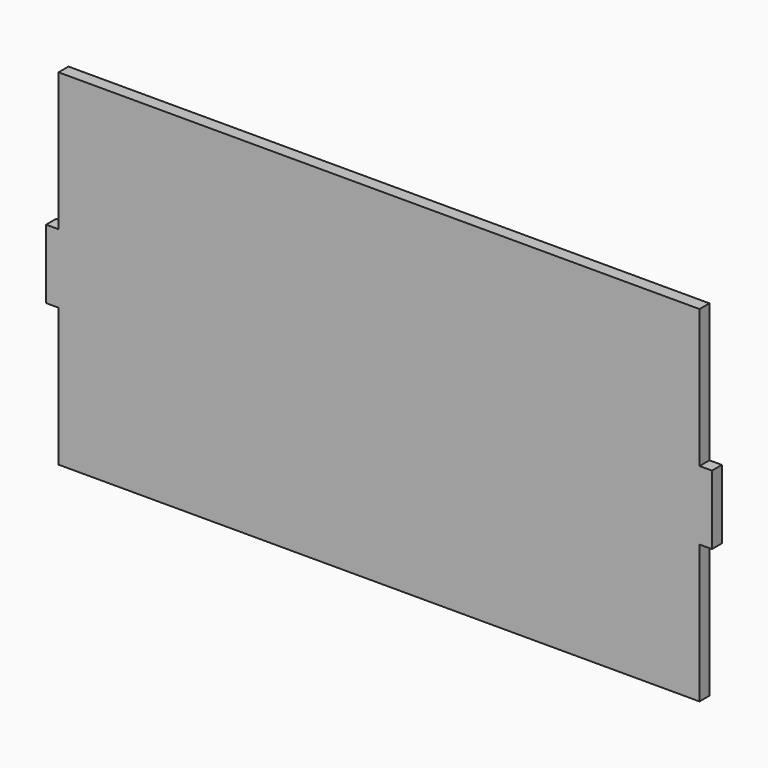
from build123d import *

# Parameters (mm, degrees)
F0_W     = 2.7432
F0_H     = 15.24
F0_W_2   = 15.24
F0_H_2   = 2.7432
F1_DEPTH = 2.7432


# Not quite as in the source:
# - a feature names something its author has since deleted; it is built from what else it names


with BuildPart() as f1:
    # F0 (on Front) → F1 (new body)
    with BuildSketch(Plane.XZ):
        Polygon((-24.1134765283, 30.4756419325), (-87.1943765283, 30.4756419325), (-87.1943765283, -0.0043580675), (-87.1943765283, -15.2443580675), (-87.1943765283, -45.7243580675), (-24.1134765283, -45.7243580675), (-24.1134765283, -42.9811580675), (-8.8734765283, -42.9811580675), (-8.8734765283, -45.7243580675), (54.2074234717, -45.7243580675), (54.2074234717, -15.2443580675), (54.2074234717, -0.0043580675), (54.2074234717, 30.4756419325), (-8.8734765283, 30.4756419325), (-8.8734765283, 27.7324419325), (-24.1134765283, 27.7324419325), align=None)
        with Locations((-88.5659765283, -7.6243580675)):
            Rectangle(F0_W, F0_H)
        with Locations((55.5790234717, -7.6243580675)):
            Rectangle(F0_W, F0_H)
        with Locations((-16.4934765283, 29.1040419325)):
            Rectangle(F0_W_2, F0_H_2)
        with Locations((-16.4934765283, -44.3527580675)):
            Rectangle(F0_W_2, F0_H_2)
    extrude(amount=F1_DEPTH)


solid = f1.part
